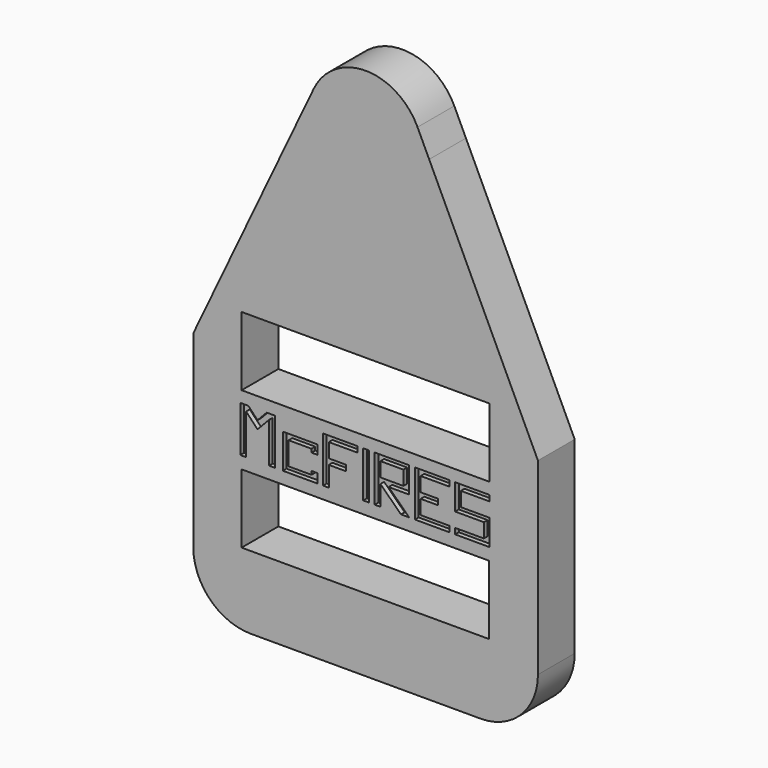
from build123d import *

# Parameters (mm, degrees)
F0_W     = 21.5146457776
F0_H     = 6
F1_DEPTH = 4
F2_W     = 0.5
F2_H     = 4
F2_W_2   = 2
F2_H_2   = 1.25
F3_DEPTH = 0.4


# Not quite as in the source:
# - a feature names something its author has since deleted; it is built from what else it names


with BuildPart() as f1:
    # F0 (on Front) → F1 (new body)
    with BuildSketch(Plane.XZ):
        with BuildLine():
            ThreePointArc((-5, 20), (0, 15), (5, 20))
            Line((5, 20), (-5, 20))
        make_face()
        with BuildLine():
            Line((-5, 20), (5, 20))
            ThreePointArc((5, 20), (4.8783151775, 21.0963763172), (4.5191835885, 22.1393876913))
            ThreePointArc((4.5191835885, 22.1393876913), (0, 25), (-4.5191835885, 22.1393876913))
            ThreePointArc((-4.5191835885, 22.1393876913), (-4.8783151775, 21.0963763172), (-5, 20))
        make_face()
        with BuildLine():
            Line((5.5319726474, 20), (5, 20))
            ThreePointArc((5, 20), (0, 15), (-5, 20))
            Line((-5, 20), (-5.5319726474, 20))
            Line((-5.5319726474, 20), (-15, 0))
            Line((-15, 0), (-10.795, 0))
            Line((-10.795, 0), (-10.795, 3))
            Line((-10.795, 3), (10.795, 3))
            Line((10.795, 3), (10.795, 0))
            Line((10.795, 0), (15, 0))
            Line((15, 0), (5.5319726474, 20))
        make_face()
        with BuildLine():
            Line((15, -16.4057657868), (15, 0))
            Line((15, 0), (10.795, 0))
            Line((10.795, 0), (10.795, -3))
            Line((10.795, -3), (-10.795, -3))
            Line((-10.795, -3), (-10.795, 0))
            Line((-10.795, 0), (-15, 0))
            Line((-15, 0), (-15, -16.4057657868))
            ThreePointArc((-15, -16.4057657868), (-13.5355339059, -19.9412996927), (-10, -21.4057657868))
            Line((-10, -21.4057657868), (10, -21.4057657868))
            ThreePointArc((10, -21.4057657868), (13.5355339059, -19.9412996927), (15, -16.4057657868))
        make_face()
        with Locations((-0.0376771112, -12.0637425241)):
            Rectangle(F0_W, F0_H, mode=Mode.SUBTRACT)
        with BuildLine():
            Line((-5.5319726474, 20), (-5, 20))
            ThreePointArc((-5, 20), (-4.8783151775, 21.0963763172), (-4.5191835885, 22.1393876913))
            Line((-4.5191835885, 22.1393876913), (-5.5319726474, 20))
        make_face()
        with BuildLine():
            ThreePointArc((4.5191835885, 22.1393876913), (4.8783151775, 21.0963763172), (5, 20))
            Line((5, 20), (5.5319726474, 20))
            Line((5.5319726474, 20), (4.5191835885, 22.1393876913))
        make_face()
    extrude(amount=F1_DEPTH)

    # F2 (on face) → F3 (cut)
    with BuildSketch(Plane.XZ.offset(4)):
        Polygon((-10.4092183411, -4.0046597868), (-10.9092183411, -4.0046597868), (-10.9092183411, -8.0046597868), (-10.4092183411, -8.0046597868), (-10.4092183411, -4.5046597868), (-10.3992183411, -4.5046597868), (-9.4092183411, -5.54676505), (-8.4192183411, -4.5046597868), (-8.4092183411, -4.5046597868), (-8.4092183411, -8.0046597868), (-7.9092183411, -8.0046597868), (-7.9092183411, -4.0046597868), (-8.4092183411, -4.0046597868), (-8.6092183411, -4.0046597868), (-9.4092183411, -4.84676505), (-10.2092183411, -4.0046597868), align=None)
        Polygon((-4.2092183411, -5.0046597868), (-7.2092183411, -5.0046597868), (-7.2092183411, -8.0046597868), (-4.2092183411, -8.0046597868), (-4.2092183411, -7.2046597868), (-4.7092183411, -7.2046597868), (-4.7092183411, -7.5046597868), (-6.7092183411, -7.5046597868), (-6.7092183411, -5.5046597868), (-4.7092183411, -5.5046597868), (-4.7092183411, -5.8046597868), (-4.2092183411, -5.8046597868), align=None)
        Polygon((-0.7092183411, -4.0046597868), (-3.7092183411, -4.0046597868), (-3.7092183411, -8.0046597868), (-3.2092183411, -8.0046597868), (-3.2092183411, -6.2546597868), (-1.7092183411, -6.2546597868), (-1.7092183411, -5.7546597868), (-3.2092183411, -5.7546597868), (-3.2092183411, -4.5046597868), (-0.7092183411, -4.5046597868), align=None)
        with Locations((0.0407816589, -6.0046597868)):
            Rectangle(F2_W, F2_H)
        Polygon((3.7907816589, -4.0046597868), (0.7907816589, -4.0046597868), (0.7907816589, -8.0046597868), (1.2907816589, -8.0046597868), (1.2907816589, -6.2546597868), (3.0764354139, -8.0046597868), (3.7907816589, -8.0046597868), (2.0051279039, -6.2546597868), (3.7907816589, -6.2546597868), align=None)
        with Locations((2.2907816589, -5.1296597868)):
            Rectangle(F2_W_2, F2_H_2, mode=Mode.SUBTRACT)
        Polygon((7.2907816589, -4.0046597868), (4.2907816589, -4.0046597868), (4.2907816589, -8.0046597868), (7.2907816589, -8.0046597868), (7.2907816589, -7.5046597868), (4.7907816589, -7.5046597868), (4.7907816589, -6.2546597868), (6.2907816589, -6.2546597868), (6.2907816589, -5.7546597868), (4.7907816589, -5.7546597868), (4.7907816589, -4.5046597868), (7.2907816589, -4.5046597868), align=None)
        Polygon((10.7907816589, -4.0046597868), (7.7907816589, -4.0046597868), (7.7907816589, -6.2546597868), (10.2907816589, -6.2546597868), (10.2907816589, -7.5046597868), (7.7907816589, -7.5046597868), (7.7907816589, -8.0046597868), (10.7907816589, -8.0046597868), (10.7907816589, -5.7546597868), (8.2907816589, -5.7546597868), (8.2907816589, -4.5046597868), (10.7907816589, -4.5046597868), align=None)
    extrude(amount=-F3_DEPTH, mode=Mode.SUBTRACT)


solid = f1.part
